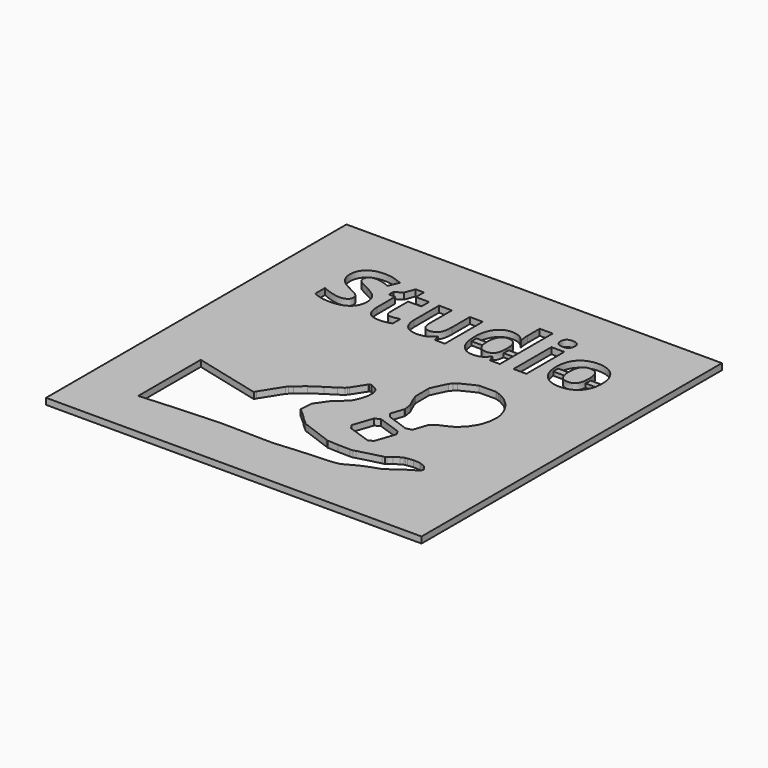
from build123d import *

# Parameters (mm, degrees)
F0_W         = 120
F0_H         = 120
F1_DEPTH     = 2
F2_TEXT_SIZE = 27.7777777778
F3_DEPTH     = 25
F5_DEPTH     = 25
F6_W         = 23.7335174595
F6_H         = 2
F7_DEPTH     = 1.2
F6_W_2       = 18.0919476534


# Not quite as in the source:
# - Text() gives the source's letters only with a copy of the font that has no kerning and outlines rounded to 1/6400 em; it was checked with that copy


with BuildPart() as f1:
    # F0 (on Top) → F1 (new body)
    with BuildSketch(Plane.XY):
        with Locations((-1, 0)):
            Rectangle(F0_W, F0_H)
    extrude(amount=F1_DEPTH)

    # F2 (on face) → F3 (cut)
    with BuildSketch(Plane.XY.offset(2)):
        with Locations((-45, 25)):
            Text('Studio', F2_TEXT_SIZE, font='Open Sans', font_style=FontStyle.BOLD, text_align=(TextAlign.LEFT, TextAlign.BOTTOM))
    extrude(amount=-F3_DEPTH, mode=Mode.SUBTRACT)

    # F4 (on face) → F5 (cut)
    with BuildSketch(Plane.XY.offset(2)):
        Polygon((-22.4251957289, -25.2047619802), (-43.6838659289, -19.8517534031), (-43.6838659289, -44.8517534031), (-40.3901329923, -44.6215304181), (-32.6644013005, -44.1226550096), (-23.7554908576, -43.6366287079), (-18.4793411572, -43.4191369478), (-16.8931248301, -43.4319860545), (-16.0426082725, -43.4319860545), (-13.4779737293, -43.4766632236), (-8.7836881633, -43.5662533253), (-4.3387224197, -43.6493599328), (-2.0875353508, -43.6749402645), (-1.6526697124, -43.6622090395), (-1.1537943039, -43.6429943203), (2.1654010826, -43.3871910036), (5.4462849126, -43.0929582485), (5.9259456018, -43.0610123044), (6.3991227969, -43.022582866), (8.6888571858, -42.9075303143), (11.2598573414, -42.7604139368), (11.8801509141, -42.7156188859), (12.7052050218, -42.6453613851), (15.9285625759, -42.5109762326), (18.4291873489, -42.1144221508), (18.8897512008, -41.9162629916), (19.1967151808, -41.7883613333), (20.8146416886, -40.9057809497), (22.7652303899, -39.850503857), (23.2385254667, -39.6458612036), (23.9165810786, -39.3387793418), (26.5643222292, -38.3347807941), (28.3741601654, -37.7080037273), (28.6428125888, -37.5864676814), (28.9048636363, -37.4585660231), (30.3120176417, -36.4417183687), (32.1283390721, -35.0538969642), (32.5951506547, -34.7468151024), (33.062080119, -34.4398511224), (35.5434901729, -32.9689231104), (36.9759887465, -31.7665296401), (36.9185803524, -31.5939508126), (36.7522492557, -31.1270213483), (35.7289181071, -29.9311113722), (33.8806507325, -29.1700670345), (31.6614096078, -29.0612622136), (29.9281947849, -29.2660227487), (29.3654274881, -29.3810753004), (29.007184963, -29.4514506829), (28.003304297, -29.9502082096), (26.5706878417, -30.8904327507), (25.4386697539, -31.7730131343), (24.9844715146, -32.1694493343), (24.2682222278, -32.2909853802), (17.2971692612, -34.1009411981), (16.619231531, -34.3438954082), (15.730285535, -34.4142707907), (11.6755082607, -34.3183150765), (8.6439442533, -34.1776821931), (8.2795718791, -34.2288428565), (7.505560553, -33.8578691064), (-0.495071293, -30.9160130824), (-1.3201254007, -30.6985213223), (-1.6270893807, -30.5002442814), (-4.313142088, -28.0954573409), (-4.5369994606, -27.8205571867), (-4.7480077264, -27.5582703757), (-7.2487503812, -25.3647274644), (-7.5366175238, -25.1920307552), (-7.2997931629, -21.1307699867), (-4.2171863738, -16.7115024565), (-3.8782764496, -16.5068598032), (-0.9044744814, -13.8976659726), (-0.6549188955, -13.5907019926), (-0.3479549154, -13.0853430899), (0.4002403156, -11.4609330879), (1.1037583774, -9.0369314281), (1.1421878158, -6.7410671901), (0.5600879181, -5.2957195098), (0.2148123814, -4.9951211422), (-0.2456335887, -4.5922014479), (-1.9723649175, -3.8118245094), (-2.6312058101, -3.9654243811), (-2.8423319577, -4.3875587946), (-5.3941173941, -8.3397789787), (-5.6947157617, -8.7045049981), (-6.1040010685, -9.1648330865), (-7.645304463, -10.2585396176), (-10.5487310486, -12.062129823), (-13.9768491378, -14.3772087802), (-16.7012134017, -16.6220302365), (-17.5134184027, -17.4598155692), (-18.0378741429, -18.0227007477), (-22.1373285863, -24.4885126934), align=None)
        Polygon((17.4827150771, -27.1106735123), (19.6506776567, -20.772763225), (18.7808284981, -19.2761369997), (11.509177164, -16.7947269458), (9.8912506561, -17.5942007218), (7.742384914, -23.9064127957), (8.74626558, -25.3390292511), (15.9541429075, -27.8078259617), align=None)
        Polygon((27.8946173579, -8.8386543872), (28.2335272821, -8.665957678), (28.9178306247, -8.2247264271), (30.7340341734, -6.5043607109), (32.5120440472, -3.7798785652), (33.4777310383, -0.678057057), (33.644062135, 1.8162021036), (33.5481064208, 2.6284071046), (33.4457850941, 3.4406121056), (32.6846228747, 5.8260664453), (31.0090522093, 8.6080748668), (28.6364469763, 10.8274338732), (26.4620009025, 12.0617732876), (25.6881074581, 12.3240600986), (24.6200991404, 12.6884324728), (19.2030807933, 12.6437553036), (14.3296150238, 10.2646665764), (13.5429903545, 9.4588271879), (12.7500000726, 8.6593534118), (10.4348032337, 3.7604251924), (10.4603835654, -1.6629587672), (10.837722928, -2.7246014725), (10.9719901989, -3.1532193801), (11.1893640772, -3.6904063452), (12.3790263225, -6.2421917816), (12.7692147918, -8.7619133922), (12.5900345884, -9.2928526265), (11.3621786681, -12.9766561507), (12.37266071, -14.4156382186), (19.4077234467, -16.8714679408), (21.1983466637, -16.3918072515), (22.4263204657, -12.6312627323), (22.6055006691, -12.0940757672), (24.594400927, -10.4312363268), (27.3380977918, -9.1711986989), align=None)
    extrude(amount=-F5_DEPTH, mode=Mode.SUBTRACT)


with BuildPart() as f7:
    # F6 (on face) → F7 (new body)
    with BuildSketch(Plane(origin=(0, 0, 0), x_dir=(1, 0, 0), z_dir=(0, 0, -1))):
        with Locations((38.2495607841, -32.3720234897)):
            Rectangle(F6_W, F6_H)
    extrude(amount=-F7_DEPTH)


with BuildPart() as f7b:
    # F6 (on face) → F7, piece 2 (new body)
    with BuildSketch(Plane(origin=(0, 0, 0), x_dir=(1, 0, 0), z_dir=(0, 0, -1))):
        with Locations((9.1622933405, -32.3720234897)):
            Rectangle(F6_W_2, F6_H)
    extrude(amount=-F7_DEPTH)


solid = Compound([f1.part, f7.part, f7b.part])
